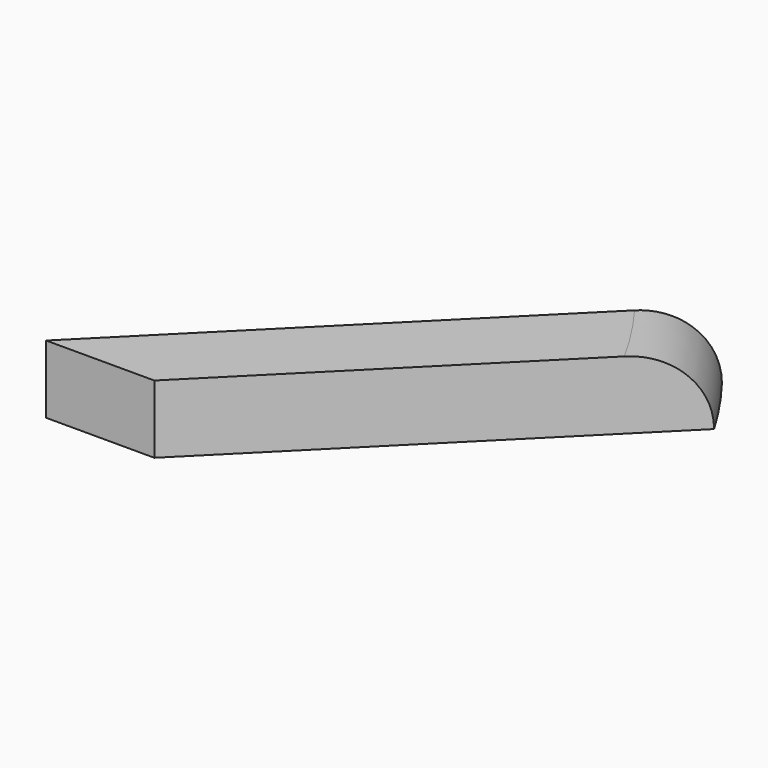
from build123d import *

# Parameters (mm, degrees)
F2_DEPTH = 25.4
F3_R     = 25.39999


# Not quite as in the source:
# - a fillet or chamfer is up to 0.001 mm smaller than in the source, because OpenCascade refuses the exact size


with BuildPart() as f2:
    # F1 (on face) → F2 (new body)
    with BuildSketch(Plane.XY):
        with BuildLine():
            Line((180.582366013, 140.1712134682), (40.4111525448, 0))
            Line((40.4111525448, 0), (80.8223050896, 0))
            Line((80.8223050896, 0), (196.9228733519, 116.1005682623))
            ThreePointArc((196.9228733519, 116.1005682623), (189.1359310844, 128.3961041965), (180.582366013, 140.1712134682))
        make_face()
    extrude(amount=F2_DEPTH)

    # F3 (radius 25.4 in the source; OpenCascade refuses exactly that, so slightly less here)
    f3_edges = [f2.edges().sort_by_distance(p)[0] for p in [
        (189.135931, 128.396104, 25.4),
    ]]
    fillet(f3_edges, radius=F3_R)


solid = f2.part
